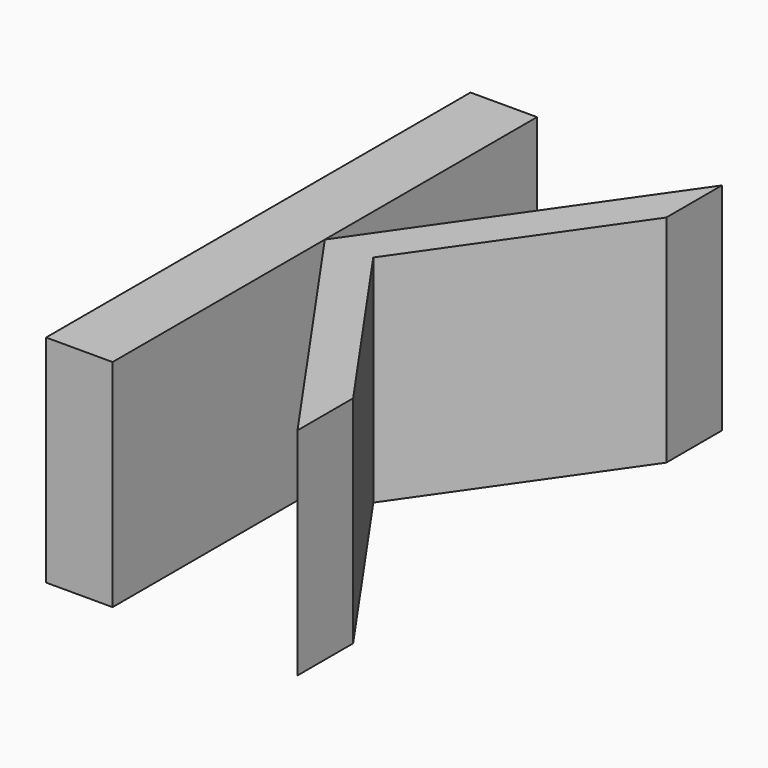
from build123d import *

# Parameters (mm, degrees)
F1_DEPTH = 25.4


# Not quite as in the source:
# - a feature of the source that left no trace in its solid (it failed there, or was rolled back) is left out


with BuildPart() as f1:
    # F0 (on Top) → F1 (new body)
    with BuildSketch(Plane.XY):
        Polygon((2.9549982864, 40.5778624117), (-18.8090335578, 9.3567771837), (2.9549982864, -21.8643080443), (2.9549982864, -13.6778589597), (-13.102308847, 9.3567771837), (2.9549982864, 32.3914133272), align=None)
    extrude(amount=F1_DEPTH)


with BuildPart() as f1b:
    # F0 (on Top) → F1, piece 2 (new body)
    with BuildSketch(Plane.XY):
        Polygon((-18.8090335578, 40.5778624117), (-26.6381744295, 40.5778624117), (-26.6381744295, -21.8643080443), (-18.8090335578, -21.8643080443), (-18.8090335578, 9.3567771837), align=None)
    extrude(amount=F1_DEPTH)


solid = Compound([f1.part, f1b.part])
